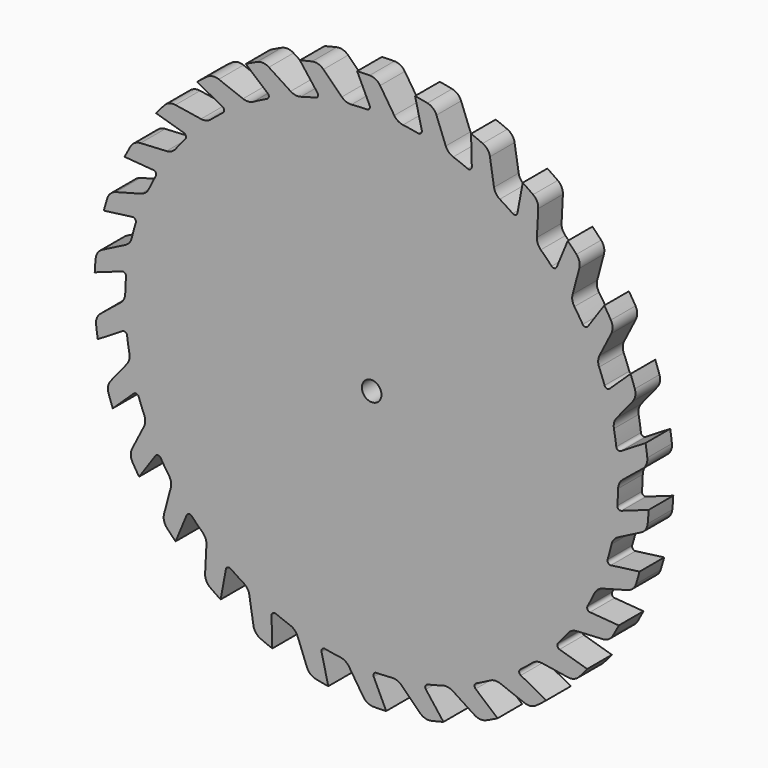
from build123d import *

# Parameters (mm, degrees)
F0_R            = 45
F1_DEPTH        = 5
F4_DEPTH        = 25
F4_COPIES_COUNT = 30
F5_R            = 2
F6_R            = 0.5
F7_R            = 1.5875
F8_DEPTH        = 25


# Not quite as in the source:
# - a pattern or mirror of a feature is missing from the dataset's text; its kind, count and spacing are read off the source's solid


with BuildPart() as f1:
    # F0 (on Front) → F1 (new body)
    with BuildSketch(Plane.XZ):
        Circle(F0_R)
    extrude(amount=F1_DEPTH)

    # F2 (on face) → F4 (cut)
    with BuildSketch(Plane.XZ.offset(5)):
        with BuildLine():
            Line((-8.5864047919, 44.1732232551), (-4.1811385307, 39.7808758147))
            ThreePointArc((-4.1811385307, 39.7808758147), (-2.0934382497, 39.9451813902), (0, 40))
            Line((0, 40), (-2.3551180309, 44.938329064))
            ThreePointArc((-2.3551180309, 44.938329064), (-5.4841204532, 44.6645768239), (-8.5864047919, 44.1732232551))
        make_face()
    f4 = extrude(amount=-F4_DEPTH, mode=Mode.SUBTRACT)

    # F4_copies: F4 ×30 about axis
    f4_copies_axis = Axis((0, 0, 0), (0, 1, 0))
    for i in range(1, F4_COPIES_COUNT):
        add(f4.rotate(f4_copies_axis, i * 360 / F4_COPIES_COUNT), mode=Mode.SUBTRACT)

    # F5
    f5_edges = [f1.edges().sort_by_distance(p)[0] for p in [
        (-8.586405, -2.5, 44.173223),
        (-4.181139, -2.5, 39.780876),
        (0.785358, -2.5, 44.993146),
        (4.181139, -2.5, 39.780876),
        (10.122797, -2.5, 43.846653),
        (12.36068, -2.5, 38.042261),
        (19.017822, -2.5, 40.78385),
        (20, -2.5, 34.641016),
        (27.081676, -2.5, 35.938598),
        (26.765224, -2.5, 29.725793),
        (33.961931, -2.5, 29.522656),
        (32.36068, -2.5, 23.51141),
        (39.357887, -2.5, 21.816433),
        (36.541818, -2.5, 16.269466),
        (43.033714, -2.5, 13.156727),
        (39.125904, -2.5, 8.316468),
        (44.828761, -2.5, 3.922008),
        (40, -2.5, 0),
        (44.664577, -2.5, -5.48412),
        (39.125904, -2.5, -8.316468),
        (42.548336, -2.5, -14.650567),
        (36.541818, -2.5, -16.269466),
        (38.572529, -2.5, -23.176713),
        (32.36068, -2.5, -23.51141),
        (32.910917, -2.5, -30.689926),
        (26.765224, -2.5, -29.725793),
        (25.81094, -2.5, -36.861842),
        (20, -2.5, -34.641016),
        (17.582901, -2.5, -41.422718),
        (12.36068, -2.5, -38.042261),
        (8.586405, -2.5, -44.173223),
        (4.181139, -2.5, -39.780876),
        (-0.785358, -2.5, -44.993146),
        (-4.181139, -2.5, -39.780876),
        (-10.122797, -2.5, -43.846653),
        (-12.36068, -2.5, -38.042261),
        (-19.017822, -2.5, -40.78385),
        (-20, -2.5, -34.641016),
        (-27.081676, -2.5, -35.938598),
        (-26.765224, -2.5, -29.725793),
        (-33.961931, -2.5, -29.522656),
        (-32.36068, -2.5, -23.51141),
        (-39.357887, -2.5, -21.816433),
        (-36.541818, -2.5, -16.269466),
        (-43.033714, -2.5, -13.156727),
        (-39.125904, -2.5, -8.316468),
        (-44.828761, -2.5, -3.922008),
        (-40, -2.5, 0),
        (-44.664577, -2.5, 5.48412),
        (-39.125904, -2.5, 8.316468),
        (-42.548336, -2.5, 14.650567),
        (-36.541818, -2.5, 16.269466),
        (-38.572529, -2.5, 23.176713),
        (-32.36068, -2.5, 23.51141),
        (-32.910917, -2.5, 30.689926),
        (-26.765224, -2.5, 29.725793),
        (-25.81094, -2.5, 36.861842),
        (-20, -2.5, 34.641016),
        (-17.582901, -2.5, 41.422718),
        (-12.36068, -2.5, 38.042261),
    ]]
    fillet(f5_edges, radius=F5_R)

    # F6
    f6_edges = [f1.edges().sort_by_distance(p)[0] for p in [
        (0, -2.5, 40),
        (-8.316468, -2.5, 39.125904),
        (8.316468, -2.5, 39.125904),
        (-16.269466, -2.5, 36.541818),
        (16.269466, -2.5, 36.541818),
        (-23.51141, -2.5, 32.36068),
        (23.51141, -2.5, 32.36068),
        (-29.725793, -2.5, 26.765224),
        (29.725793, -2.5, 26.765224),
        (-34.641016, -2.5, 20),
        (34.641016, -2.5, 20),
        (-38.042261, -2.5, 12.36068),
        (38.042261, -2.5, 12.36068),
        (-39.780876, -2.5, 4.181139),
        (39.780876, -2.5, 4.181139),
        (-39.780876, -2.5, -4.181139),
        (39.780876, -2.5, -4.181139),
        (-38.042261, -2.5, -12.36068),
        (38.042261, -2.5, -12.36068),
        (-34.641016, -2.5, -20),
        (34.641016, -2.5, -20),
        (-29.725793, -2.5, -26.765224),
        (29.725793, -2.5, -26.765224),
        (-23.51141, -2.5, -32.36068),
        (23.51141, -2.5, -32.36068),
        (-16.269466, -2.5, -36.541818),
        (16.269466, -2.5, -36.541818),
        (-8.316468, -2.5, -39.125904),
        (8.316468, -2.5, -39.125904),
        (0, -2.5, -40),
    ]]
    fillet(f6_edges, radius=F6_R)

    # F7 (on face) → F8 (cut)
    with BuildSketch(Plane.XZ.offset(5)):
        Circle(F7_R)
    extrude(amount=-F8_DEPTH, mode=Mode.SUBTRACT)


solid = f1.part
